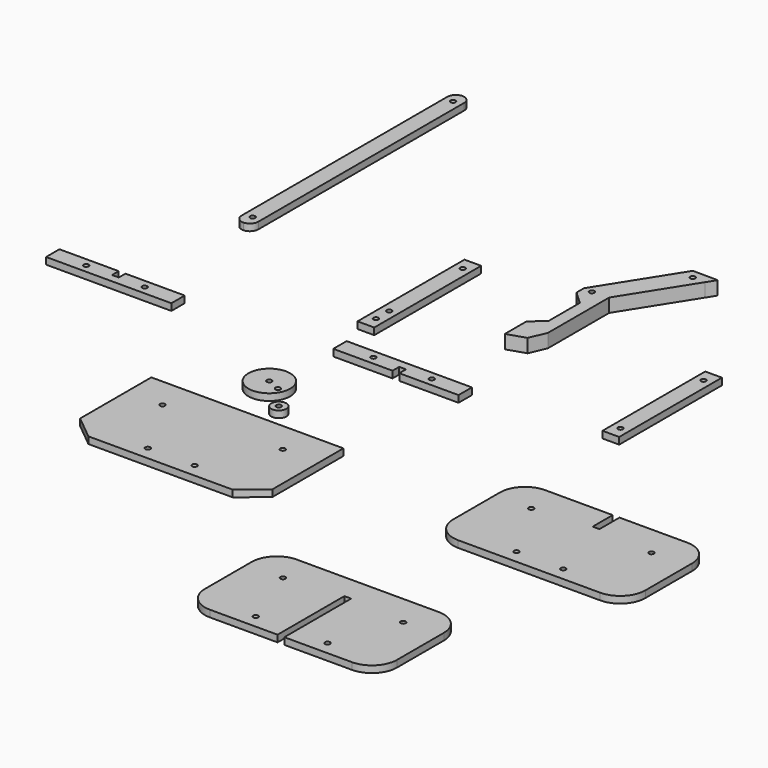
from build123d import *

# Parameters (mm, degrees)
F1_DEPTH = 8.128
F2_R     = 1.5
F3_DEPTH = 4.064
F2_R_2   = 12.5
F2_R_3   = 4.5
F4_R     = 4.99999
F5_R     = 4.99999
F6_R     = 15
F7_R     = 15


# Not quite as in the source:
# - a fillet or chamfer is up to 0.001 mm smaller than in the source, because OpenCascade refuses the exact size
# - a feature names something its author has since deleted; it is built from what else it names


with BuildPart() as f1:
    # F0 (on Top) → F1 (new body)
    with BuildSketch(Plane.XY):
        with BuildLine():
            Line((25.3375305185, 90.8126524978), (0, 50.6579922774))
            Line((0, 50.6579922774), (0, 50.0453769267))
            Line((0, 50.0453769267), (3.6980586722, 50.0453769267))
            ThreePointArc((3.6980586722, 50.0453769267), (5.1980586722, 51.5453769267), (6.6980586722, 50.0453769267))
            Line((6.6980586722, 50.0453769267), (15.0774987414, 50.0453769267))
            Line((15.0774987414, 50.0453769267), (15.0774987414, 50.6579922774))
            Line((15.0774987414, 50.6579922774), (40.41502926, 90.8126524978))
            Line((40.41502926, 90.8126524978), (34.3762798892, 90.8126524978))
            ThreePointArc((34.3762798892, 90.8126524978), (32.8762798892, 89.3126524978), (31.3762798892, 90.8126524978))
            Line((31.3762798892, 90.8126524978), (25.3375305185, 90.8126524978))
        make_face()
        with BuildLine():
            Line((3.6980586722, 50.0453769267), (0, 50.0453769267))
            Line((0, 50.0453769267), (0, 45.0453769267))
            Line((0, 45.0453769267), (7.7709886245, 45.0453769267))
            Line((7.7709886245, 45.0453769267), (7.7709886245, 37.8160925433))
            Line((7.7709886245, 37.8160925433), (7.7709886245, 26.2229798213))
            Line((7.7709886245, 26.2229798213), (7.7709886245, 14.6298670992))
            Line((7.7709886245, 14.6298670992), (7.7709886245, 7.4005827159))
            Line((7.7709886245, 7.4005827159), (0, 7.4005827159))
            Line((0, 7.4005827159), (0, -8.5994172841))
            Line((0, -8.5994172841), (10.7996687293, -5.1236809231))
            Line((10.7996687293, -5.1236809231), (15.0774987414, 4.7687999904))
            Line((15.0774987414, 4.7687999904), (15.0774987414, 50.0453769267))
            Line((15.0774987414, 50.0453769267), (6.6980586722, 50.0453769267))
            ThreePointArc((6.6980586722, 50.0453769267), (5.1980586722, 48.5453769267), (3.6980586722, 50.0453769267))
        make_face()
        with BuildLine():
            Line((28.7261359414, 96.182879848), (25.3375305185, 90.8126524978))
            Line((25.3375305185, 90.8126524978), (31.3762798892, 90.8126524978))
            ThreePointArc((31.3762798892, 90.8126524978), (32.8762798892, 92.3126524978), (34.3762798892, 90.8126524978))
            Line((34.3762798892, 90.8126524978), (40.41502926, 90.8126524978))
            Line((40.41502926, 90.8126524978), (43.7256264815, 96.0592532453))
            Line((43.7256264815, 96.0592532453), (28.7261359414, 96.182879848))
        make_face()
        Polygon((7.7709886245, 45.0453769267), (0, 45.0453769267), (7.7709886245, 37.8160925433), align=None)
        Polygon((7.7709886245, 7.4005827159), (7.7709886245, 14.6298670992), (0, 7.4005827159), align=None)
    extrude(amount=F1_DEPTH)


with BuildPart() as f3:
    # F2 (on Top) → F3 (new body)
    with BuildSketch(Plane.XY):
        Polygon((-92.1053215861, -140.0898771882), (-106.4274155871, -140.0898771882), (-106.4274155871, -151.8304497004), align=None)
        Polygon((8.5725844129, -140.0898771882), (-5.7495095881, -140.0898771882), (8.5725844129, -151.8304497004), align=None)
        Polygon((-48.9274155871, -140.0898771882), (-92.1053215861, -140.0898771882), (-106.4274155871, -151.8304497004), (-106.4274155871, -172.5898771882), (-48.9274155871, -172.5898771882), align=None)
        with Locations((-84.9274155871, -158.5898771882)):
            Circle(F2_R, mode=Mode.SUBTRACT)
        Polygon((-48.9274155871, -172.5898771882), (-106.4274155871, -172.5898771882), (-106.4274155871, -193.3493046761), (-92.1053215861, -205.0898771882), (-48.9274155871, -205.0898771882), align=None)
        with Locations((-62.9274155871, -197.0898771882)):
            Circle(F2_R, mode=Mode.SUBTRACT)
        Polygon((-5.7495095881, -140.0898771882), (-48.9274155871, -140.0898771882), (-48.9274155871, -172.5898771882), (8.5725844129, -172.5898771882), (8.5725844129, -151.8304497004), align=None)
        with Locations((-12.9274155871, -158.5898771882)):
            Circle(F2_R, mode=Mode.SUBTRACT)
        Polygon((8.5725844129, -172.5898771882), (-48.9274155871, -172.5898771882), (-48.9274155871, -205.0898771882), (-5.7495095881, -205.0898771882), (8.5725844129, -193.3493046761), align=None)
        with Locations((-34.9274155871, -197.0898771882)):
            Circle(F2_R, mode=Mode.SUBTRACT)
    extrude(amount=F3_DEPTH)


with BuildPart() as f3b:
    # F2 (on Top) → F3, piece 2 (new body)
    with BuildSketch(Plane.XY):
        with BuildLine():
            Line((-56.5896742046, 44.4182286735), (-66.5896742046, 44.4182286735))
            Line((-66.5896742046, 44.4182286735), (-66.5896742046, -18.1863000616))
            Line((-66.5896742046, -18.1863000616), (-63.0896742046, -18.1863000616))
            ThreePointArc((-63.0896742046, -18.1863000616), (-61.5896742046, -16.6863000616), (-60.0896742046, -18.1863000616))
            Line((-60.0896742046, -18.1863000616), (-56.5896742046, -18.1863000616))
            Line((-56.5896742046, -18.1863000616), (-56.5896742046, 44.4182286735))
        make_face()
        with Locations((-61.5896742046, 36.9182286735)):
            Circle(F2_R, mode=Mode.SUBTRACT)
        with BuildLine():
            Line((-63.0896742046, -18.1863000616), (-66.5896742046, -18.1863000616))
            Line((-66.5896742046, -18.1863000616), (-66.5896742046, -35.5817713265))
            Line((-66.5896742046, -35.5817713265), (-56.5896742046, -35.5817713265))
            Line((-56.5896742046, -35.5817713265), (-56.5896742046, -18.1863000616))
            Line((-56.5896742046, -18.1863000616), (-60.0896742046, -18.1863000616))
            ThreePointArc((-60.0896742046, -18.1863000616), (-61.5896742046, -19.6863000616), (-63.0896742046, -18.1863000616))
        make_face()
        with Locations((-61.5896742046, -28.0817713265)):
            Circle(F2_R, mode=Mode.SUBTRACT)
    extrude(amount=F3_DEPTH)


with BuildPart() as f3c:
    # F2 (on Top) → F3, piece 3 (new body)
    with BuildSketch(Plane.XY):
        with Locations((-61.0836856067, -108.4747463465)):
            Circle(F2_R_2)
        with Locations((-61.0836856067, -108.4747463465)):
            Circle(F2_R, mode=Mode.SUBTRACT)
        with Locations((-53.1394029407, -111.9610396974)):
            Circle(F2_R, mode=Mode.SUBTRACT)
    extrude(amount=F3_DEPTH)


with BuildPart() as f3d:
    # F2 (on Top) → F3, piece 4 (new body)
    with BuildSketch(Plane.XY):
        with BuildLine():
            Line((102.0343697071, 18.8202806036), (98.5343697071, 18.8202806036))
            ThreePointArc((98.5343697071, 18.8202806036), (97.0343697071, 17.3202806036), (95.5343697071, 18.8202806036))
            Line((95.5343697071, 18.8202806036), (92.0343697071, 18.8202806036))
            Line((92.0343697071, 18.8202806036), (92.0343697071, -43.3527193964))
            Line((92.0343697071, -43.3527193964), (95.5343697071, -43.3527193964))
            ThreePointArc((95.5343697071, -43.3527193964), (97.0343697071, -41.8527193964), (98.5343697071, -43.3527193964))
            Line((98.5343697071, -43.3527193964), (102.0343697071, -43.3527193964))
            Line((102.0343697071, -43.3527193964), (102.0343697071, 18.8202806036))
        make_face()
        with BuildLine():
            ThreePointArc((95.5343697071, 18.8202806036), (97.0343697071, 20.3202806036), (98.5343697071, 18.8202806036))
            Line((98.5343697071, 18.8202806036), (102.0343697071, 18.8202806036))
            Line((102.0343697071, 18.8202806036), (102.0343697071, 26.3015180826))
            Line((102.0343697071, 26.3015180826), (92.0343697071, 26.3015180826))
            Line((92.0343697071, 26.3015180826), (92.0343697071, 18.8202806036))
            Line((92.0343697071, 18.8202806036), (95.5343697071, 18.8202806036))
        make_face()
        with BuildLine():
            Line((102.0343697071, -50.5698025227), (102.0343697071, -43.3527193964))
            Line((102.0343697071, -43.3527193964), (98.5343697071, -43.3527193964))
            ThreePointArc((98.5343697071, -43.3527193964), (97.0343697071, -44.8527193964), (95.5343697071, -43.3527193964))
            Line((95.5343697071, -43.3527193964), (92.0343697071, -43.3527193964))
            Line((92.0343697071, -43.3527193964), (92.0343697071, -50.5698025227))
            Line((92.0343697071, -50.5698025227), (102.0343697071, -50.5698025227))
        make_face()
    extrude(amount=F3_DEPTH)


with BuildPart() as f3e:
    # F2 (on Top) → F3, piece 5 (new body)
    with BuildSketch(Plane.XY):
        with Locations((-41.755348444, -125.5374103785)):
            Circle(F2_R_3)
        with Locations((-41.755348444, -125.5374103785)):
            Circle(F2_R, mode=Mode.SUBTRACT)
    extrude(amount=F3_DEPTH)


with BuildPart() as f3f:
    # F2 (on Top) → F3, piece 6 (new body)
    with BuildSketch(Plane.XY):
        with BuildLine():
            Line((-20.5745910993, -54.3875524402), (-38.0745910993, -54.3875524402))
            Line((-38.0745910993, -54.3875524402), (-38.0745910993, -57.8875524402))
            ThreePointArc((-38.0745910993, -57.8875524402), (-37.0139309275, -58.3268922684), (-36.5745910993, -59.3875524402))
            ThreePointArc((-36.5745910993, -59.3875524402), (-37.0139309275, -60.4482126119), (-38.0745910993, -60.8875524402))
            Line((-38.0745910993, -60.8875524402), (-38.0745910993, -64.3875524402))
            Line((-38.0745910993, -64.3875524402), (-22.6065910993, -64.3875524402))
            Line((-22.6065910993, -64.3875524402), (-22.6065910993, -59.3875524402))
            Line((-22.6065910993, -59.3875524402), (-20.5745910993, -59.3875524402))
            Line((-20.5745910993, -59.3875524402), (-20.5745910993, -54.3875524402))
        make_face()
        with BuildLine():
            Line((-38.0745910993, -54.3875524402), (-58.0745910993, -54.3875524402))
            Line((-58.0745910993, -54.3875524402), (-58.0745910993, -64.3875524402))
            Line((-58.0745910993, -64.3875524402), (-38.0745910993, -64.3875524402))
            Line((-38.0745910993, -64.3875524402), (-38.0745910993, -60.8875524402))
            ThreePointArc((-38.0745910993, -60.8875524402), (-39.5745910993, -59.3875524402), (-38.0745910993, -57.8875524402))
            Line((-38.0745910993, -57.8875524402), (-38.0745910993, -54.3875524402))
        make_face()
        with BuildLine():
            Line((16.9254089007, -54.3875524402), (-3.0745910993, -54.3875524402))
            Line((-3.0745910993, -54.3875524402), (-3.0745910993, -57.8875524402))
            ThreePointArc((-3.0745910993, -57.8875524402), (-2.0139309275, -58.3268922684), (-1.5745910993, -59.3875524402))
            ThreePointArc((-1.5745910993, -59.3875524402), (-2.0139309275, -60.4482126119), (-3.0745910993, -60.8875524402))
            Line((-3.0745910993, -60.8875524402), (-3.0745910993, -64.3875524402))
            Line((-3.0745910993, -64.3875524402), (16.9254089007, -64.3875524402))
            Line((16.9254089007, -64.3875524402), (16.9254089007, -54.3875524402))
        make_face()
        with BuildLine():
            Line((-3.0745910993, -54.3875524402), (-20.5745910993, -54.3875524402))
            Line((-20.5745910993, -54.3875524402), (-20.5745910993, -59.3875524402))
            Line((-20.5745910993, -59.3875524402), (-18.5425910993, -59.3875524402))
            Line((-18.5425910993, -59.3875524402), (-18.5425910993, -64.3875524402))
            Line((-18.5425910993, -64.3875524402), (-3.0745910993, -64.3875524402))
            Line((-3.0745910993, -64.3875524402), (-3.0745910993, -60.8875524402))
            ThreePointArc((-3.0745910993, -60.8875524402), (-4.5745910993, -59.3875524402), (-3.0745910993, -57.8875524402))
            Line((-3.0745910993, -57.8875524402), (-3.0745910993, -54.3875524402))
        make_face()
    extrude(amount=F3_DEPTH)


with BuildPart() as f3g:
    # F2 (on Top) → F3, piece 7 (new body)
    with BuildSketch(Plane.XY):
        with BuildLine():
            Line((-165.816038847, 166.2015340924), (-169.316038847, 166.2015340924))
            ThreePointArc((-169.316038847, 166.2015340924), (-170.816038847, 164.7015340924), (-172.316038847, 166.2015340924))
            Line((-172.316038847, 166.2015340924), (-175.816038847, 166.2015340924))
            Line((-175.816038847, 166.2015340924), (-175.816038847, 16.2015340924))
            Line((-175.816038847, 16.2015340924), (-172.316038847, 16.2015340924))
            ThreePointArc((-172.316038847, 16.2015340924), (-170.816038847, 17.7015340924), (-169.316038847, 16.2015340924))
            Line((-169.316038847, 16.2015340924), (-165.816038847, 16.2015340924))
            Line((-165.816038847, 16.2015340924), (-165.816038847, 166.2015340924))
        make_face()
        with BuildLine():
            ThreePointArc((-172.316038847, 166.2015340924), (-170.816038847, 167.7015340924), (-169.316038847, 166.2015340924))
            Line((-169.316038847, 166.2015340924), (-165.816038847, 166.2015340924))
            Line((-165.816038847, 166.2015340924), (-165.816038847, 173.2015340924))
            Line((-165.816038847, 173.2015340924), (-175.816038847, 173.2015340924))
            Line((-175.816038847, 173.2015340924), (-175.816038847, 166.2015340924))
            Line((-175.816038847, 166.2015340924), (-172.316038847, 166.2015340924))
        make_face()
        with BuildLine():
            Line((-165.816038847, 9.2015340924), (-165.816038847, 16.2015340924))
            Line((-165.816038847, 16.2015340924), (-169.316038847, 16.2015340924))
            ThreePointArc((-169.316038847, 16.2015340924), (-170.816038847, 14.7015340924), (-172.316038847, 16.2015340924))
            Line((-172.316038847, 16.2015340924), (-175.816038847, 16.2015340924))
            Line((-175.816038847, 16.2015340924), (-175.816038847, 9.2015340924))
            Line((-175.816038847, 9.2015340924), (-165.816038847, 9.2015340924))
        make_face()
    extrude(amount=F3_DEPTH)

    # F4 (radius 5 in the source; OpenCascade refuses exactly that, so slightly less here)
    f4_edges = [f3g.edges().sort_by_distance(p)[0] for p in [
        (-165.816039, 9.201534, 2.032),
        (-175.816039, 9.201534, 2.032),
    ]]
    fillet(f4_edges, radius=F4_R)

    # F5 (radius 5 in the source; OpenCascade refuses exactly that, so slightly less here)
    f5_edges = [f3g.edges().sort_by_distance(p)[0] for p in [
        (-165.816039, 173.201534, 2.032),
        (-175.816039, 173.201534, 2.032),
    ]]
    fillet(f5_edges, radius=F5_R)


with BuildPart() as f3h:
    # F2 (on Top) → F3, piece 8 (new body)
    with BuildSketch(Plane.XY):
        Polygon((149.0594564133, -114.2240408659), (107.9135504143, -114.2240408659), (93.5914564133, -125.964613378), (93.5914564133, -146.7240408659), (151.0914564133, -146.7240408659), (151.0914564133, -129.2240408659), (149.0594564133, -129.2240408659), align=None)
        with Locations((115.0914564133, -132.7240408659)):
            Circle(F2_R, mode=Mode.SUBTRACT)
        Polygon((151.0914564133, -146.7240408659), (93.5914564133, -146.7240408659), (93.5914564133, -167.4834683537), (107.9135504143, -179.2240408659), (151.0914564133, -179.2240408659), align=None)
        with Locations((137.0914564133, -171.2240408659)):
            Circle(F2_R, mode=Mode.SUBTRACT)
        Polygon((208.5914564133, -146.7240408659), (151.0914564133, -146.7240408659), (151.0914564133, -179.2240408659), (194.2693624123, -179.2240408659), (208.5914564133, -167.4834683537), align=None)
        with Locations((165.0914564133, -171.2240408659)):
            Circle(F2_R, mode=Mode.SUBTRACT)
        Polygon((151.0914564133, -129.2240408659), (151.0914564133, -146.7240408659), (208.5914564133, -146.7240408659), (208.5914564133, -125.964613378), (194.2693624123, -114.2240408659), (153.1234564133, -114.2240408659), (153.1234564133, -129.2240408659), align=None)
        with Locations((187.0914564133, -132.7240408659)):
            Circle(F2_R, mode=Mode.SUBTRACT)
        Polygon((208.5914564133, -114.2240408659), (194.2693624123, -114.2240408659), (208.5914564133, -125.964613378), align=None)
        Polygon((107.9135504143, -114.2240408659), (93.5914564133, -114.2240408659), (93.5914564133, -125.964613378), align=None)
        Polygon((107.9135504143, -179.2240408659), (93.5914564133, -167.4834683537), (93.5914564133, -179.2240408659), align=None)
        Polygon((208.5914564133, -167.4834683537), (194.2693624123, -179.2240408659), (208.5914564133, -179.2240408659), align=None)
    extrude(amount=F3_DEPTH)

    # F7
    f7_edges = [f3h.edges().sort_by_distance(p)[0] for p in [
        (93.591456, -179.224041, 2.032),
        (208.591456, -179.224041, 2.032),
        (208.591456, -114.224041, 2.032),
        (93.591456, -114.224041, 2.032),
    ]]
    fillet(f7_edges, radius=F7_R)


with BuildPart() as f3i:
    # F2 (on Top) → F3, piece 9 (new body)
    with BuildSketch(Plane.XY):
        Polygon((161.903115809, -294.9013158679), (161.903115809, -274.1418883801), (106.435115809, -274.1418883801), (106.435115809, -306.6418883801), (147.581021808, -306.6418883801), align=None)
        with Locations((125.903115809, -298.6418883801)):
            Circle(F2_R, mode=Mode.SUBTRACT)
        Polygon((147.581021808, -241.6418883801), (104.403115809, -241.6418883801), (104.403115809, -256.6418883801), (106.435115809, -256.6418883801), (106.435115809, -274.1418883801), (161.903115809, -274.1418883801), (161.903115809, -253.3824608922), align=None)
        with Locations((140.403115809, -260.1418883801)):
            Circle(F2_R, mode=Mode.SUBTRACT)
        Polygon((161.903115809, -241.6418883801), (147.581021808, -241.6418883801), (161.903115809, -253.3824608922), align=None)
        Polygon((161.903115809, -306.6418883801), (161.903115809, -294.9013158679), (147.581021808, -306.6418883801), align=None)
        Polygon((102.371115809, -274.1418883801), (46.903115809, -274.1418883801), (46.903115809, -294.9013158679), (61.22520981, -306.6418883801), (102.371115809, -306.6418883801), align=None)
        with Locations((82.903115809, -298.6418883801)):
            Circle(F2_R, mode=Mode.SUBTRACT)
        Polygon((61.22520981, -306.6418883801), (46.903115809, -294.9013158679), (46.903115809, -306.6418883801), align=None)
        Polygon((104.403115809, -241.6418883801), (61.22520981, -241.6418883801), (46.903115809, -253.3824608922), (46.903115809, -274.1418883801), (102.371115809, -274.1418883801), (102.371115809, -256.6418883801), (104.403115809, -256.6418883801), align=None)
        with Locations((68.403115809, -260.1418883801)):
            Circle(F2_R, mode=Mode.SUBTRACT)
        Polygon((61.22520981, -241.6418883801), (46.903115809, -241.6418883801), (46.903115809, -253.3824608922), align=None)
    extrude(amount=F3_DEPTH)

    # F6
    f6_edges = [f3i.edges().sort_by_distance(p)[0] for p in [
        (46.903116, -241.641888, 2.032),
        (46.903116, -306.641888, 2.032),
        (161.903116, -241.641888, 2.032),
        (161.903116, -306.641888, 2.032),
    ]]
    fillet(f6_edges, radius=F6_R)


with BuildPart() as f3j:
    # F2 (on Top) → F3, piece 10 (new body)
    with BuildSketch(Plane.XY):
        with BuildLine():
            Line((-200.9884732962, -65.641502738), (-220.9884732962, -65.641502738))
            Line((-220.9884732962, -65.641502738), (-220.9884732962, -75.641502738))
            Line((-220.9884732962, -75.641502738), (-200.9884732962, -75.641502738))
            Line((-200.9884732962, -75.641502738), (-200.9884732962, -72.141502738))
            ThreePointArc((-200.9884732962, -72.141502738), (-202.4884732962, -70.641502738), (-200.9884732962, -69.141502738))
            Line((-200.9884732962, -69.141502738), (-200.9884732962, -65.641502738))
        make_face()
        with BuildLine():
            Line((-185.5204732962, -65.641502738), (-200.9884732962, -65.641502738))
            Line((-200.9884732962, -65.641502738), (-200.9884732962, -69.141502738))
            ThreePointArc((-200.9884732962, -69.141502738), (-199.9278131244, -69.5808425662), (-199.4884732962, -70.641502738))
            ThreePointArc((-199.4884732962, -70.641502738), (-199.9278131244, -71.7021629098), (-200.9884732962, -72.141502738))
            Line((-200.9884732962, -72.141502738), (-200.9884732962, -75.641502738))
            Line((-200.9884732962, -75.641502738), (-183.4884732962, -75.641502738))
            Line((-183.4884732962, -75.641502738), (-183.4884732962, -70.641502738))
            Line((-183.4884732962, -70.641502738), (-185.5204732962, -70.641502738))
            Line((-185.5204732962, -70.641502738), (-185.5204732962, -65.641502738))
        make_face()
        with BuildLine():
            Line((-183.4884732962, -70.641502738), (-183.4884732962, -75.641502738))
            Line((-183.4884732962, -75.641502738), (-165.9884732962, -75.641502738))
            Line((-165.9884732962, -75.641502738), (-165.9884732962, -72.141502738))
            ThreePointArc((-165.9884732962, -72.141502738), (-167.4884732962, -70.641502738), (-165.9884732962, -69.141502738))
            Line((-165.9884732962, -69.141502738), (-165.9884732962, -65.641502738))
            Line((-165.9884732962, -65.641502738), (-181.4564732962, -65.641502738))
            Line((-181.4564732962, -65.641502738), (-181.4564732962, -70.641502738))
            Line((-181.4564732962, -70.641502738), (-183.4884732962, -70.641502738))
        make_face()
        with BuildLine():
            Line((-165.9884732962, -72.141502738), (-165.9884732962, -75.641502738))
            Line((-165.9884732962, -75.641502738), (-145.9884732962, -75.641502738))
            Line((-145.9884732962, -75.641502738), (-145.9884732962, -65.641502738))
            Line((-145.9884732962, -65.641502738), (-165.9884732962, -65.641502738))
            Line((-165.9884732962, -65.641502738), (-165.9884732962, -69.141502738))
            ThreePointArc((-165.9884732962, -69.141502738), (-164.9278131244, -69.5808425662), (-164.4884732962, -70.641502738))
            ThreePointArc((-164.4884732962, -70.641502738), (-164.9278131244, -71.7021629098), (-165.9884732962, -72.141502738))
        make_face()
    extrude(amount=F3_DEPTH)


solid = Compound([f1.part, f3.part, f3b.part, f3c.part, f3d.part, f3e.part, f3f.part, f3g.part, f3h.part, f3i.part, f3j.part])
